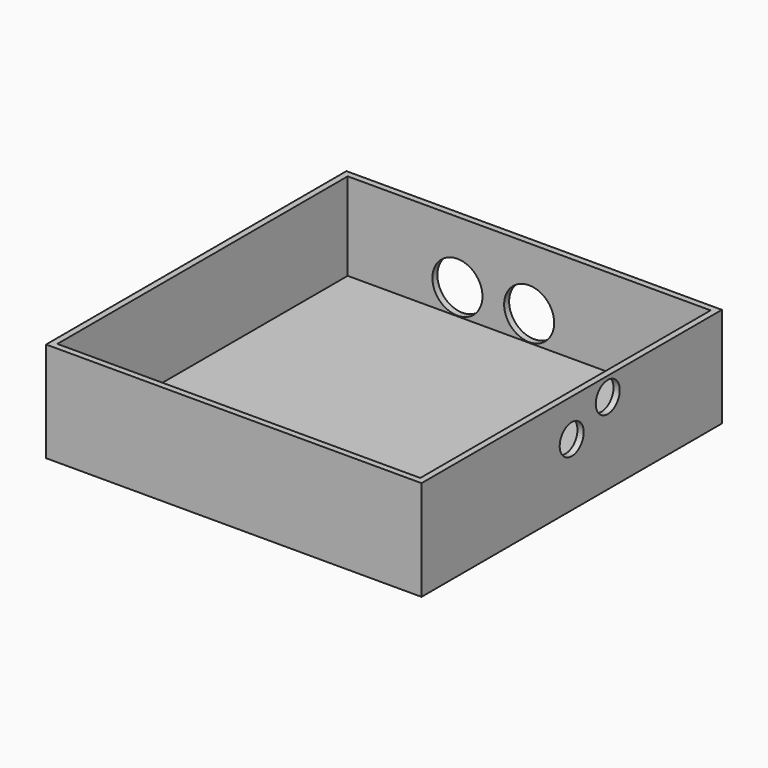
from build123d import *

# Parameters (mm, degrees)
F0_W      = 150
F0_H      = 150
F1_DEPTH  = 40
F2_W      = 145
F2_H      = 145
F3_DEPTH  = 135
F6_D      = 20
F6_DEPTH  = 5
F6_TIP    = 6.0086061903
F7_W      = 150
F7_H      = 150
F8_DEPTH  = 5
F10_D     = 12
F10_DEPTH = 5
F10_TIP   = 3.6051637142


with BuildPart() as f1:
    # F0 (on Top) → F1 (new body)
    with BuildSketch(Plane.XY):
        with Locations((39.0263837129, 41.0243682017)):
            Rectangle(F0_W, F0_H)
    extrude(amount=F1_DEPTH)

    # F2 (on face) → F3 (cut)
    with BuildSketch(Plane.XY.offset(40)):
        with Locations((39.0263837129, 41.0243682017)):
            Rectangle(F2_W, F2_H)
    extrude(amount=-F3_DEPTH, mode=Mode.SUBTRACT)

    # F6
    with Locations(Plane(origin=(0, 116.0243682017, 0), x_dir=(-1, 0, 0), z_dir=(0, 1, 0))):
        with Locations((-39.0263837129, 15.2529580519), (-10.3633506224, 15.2529580519)):
            Hole(F6_D / 2, depth=F6_DEPTH)
            with Locations((0, 0, -(F6_DEPTH + F6_TIP / 2))):  # 118° drill point
                Cone(0, F6_D / 2, F6_TIP, mode=Mode.SUBTRACT)

    # F7 (on Top) → F8 (join)
    with BuildSketch(Plane.XY):
        with Locations((38.9731861651, 41.1050692201)):
            Rectangle(F7_W, F7_H)
    extrude(amount=F8_DEPTH)

    # F10
    with Locations(Plane.YZ.offset(114.0263837129)):
        with Locations((59.0243682017, 32.5), (41.0243682017, 25)):
            Hole(F10_D / 2, depth=F10_DEPTH)
            with Locations((0, 0, -(F10_DEPTH + F10_TIP / 2))):  # 118° drill point
                Cone(0, F10_D / 2, F10_TIP, mode=Mode.SUBTRACT)


solid = f1.part
